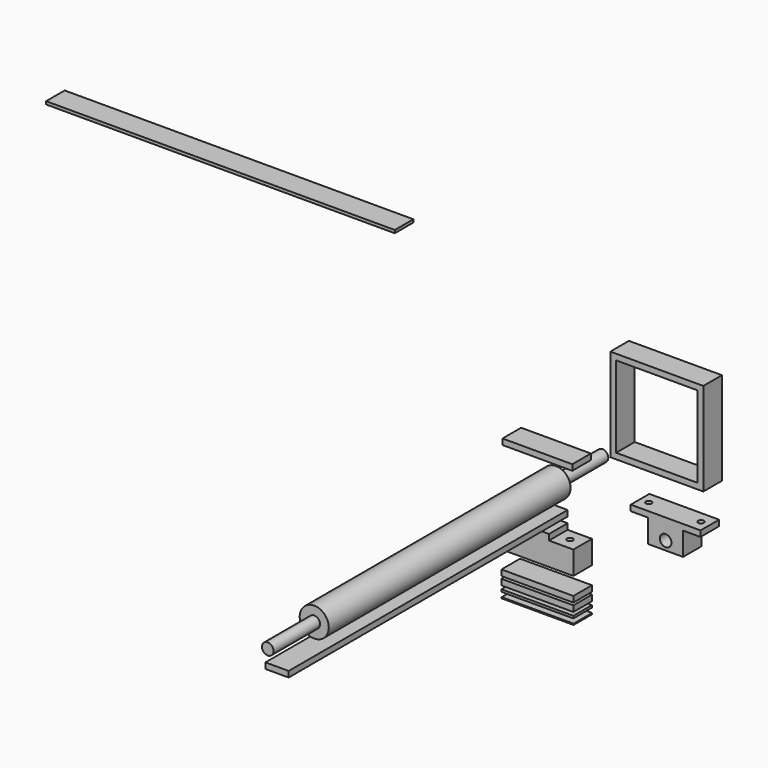
from build123d import *

# Parameters (mm, degrees)
F0_R      = 5
F1_DEPTH  = 20
F0_W      = 60
F0_H      = 5
F0_W_2    = 80
F0_H_2    = 80
F0_W_3    = 70
F0_H_3    = 70
F0_W_4    = 61.861140081
F0_H_4    = 1
F0_H_5    = 2
F0_W_5    = 300
F0_H_6    = 2.5
F0_R_2    = 12.5
F2_DEPTH  = 260
F3_R      = 5
F4_DEPTH  = 50
F5_DEPTH  = 300
F6_R      = 2.5
F7_R      = 2.5
F8_DEPTH  = 25
F10_R     = 2.5
F9_R      = 2.5
F11_DEPTH = 25
F17_R     = 5
F18_DEPTH = 50


# Not quite as in the source:
# - a feature of the source that left no trace in its solid (it failed there, or was rolled back) is left out
# - a feature names something its author has since deleted; it is built from what else it names


with BuildPart() as f1:
    # F0 (on Front) → F1 (new body)
    with BuildSketch(Plane.XZ):
        Polygon((95.2936565876, -7.5), (110.2936565876, -7.5), (125.2936565876, -7.5), (125.2936565876, 12.5), (140.2936565876, 12.5), (140.2936565876, 17.5), (110.2936565876, 17.5), (80.2936565876, 17.5), (80.2936565876, 12.5), (95.2936565876, 12.5), align=None)
        with Locations((110.2936565876, 0)):
            Circle(F0_R, mode=Mode.SUBTRACT)
    extrude(amount=F1_DEPTH)

    # F10 (on face) + F9 (on face) → F11 (cut)
    with BuildSketch(Plane(origin=(0, 0, 12.5), x_dir=(1, 0, 0), z_dir=(0, 0, -1))):
        with Locations((87.7936565876, 10)):
            Circle(F10_R)
    with BuildSketch(Plane(origin=(0, 0, 12.5), x_dir=(1, 0, 0), z_dir=(0, 0, -1))):
        with Locations((132.7936565876, 10)):
            Circle(F9_R)
    extrude(amount=-F11_DEPTH, mode=Mode.SUBTRACT)


with BuildPart() as f1b:
    # F0 (on Front) → F1, piece 2 (new body)
    with BuildSketch(Plane.XZ):
        with Locations((0, 29.2427036911)):
            Rectangle(F0_W, F0_H)
    extrude(amount=F1_DEPTH)


with BuildPart() as f1c:
    # F0 (on Front) → F1, piece 3 (new body)
    with BuildSketch(Plane.XZ):
        Polygon((10, -27.5771580637), (0, -27.5771580637), (-10, -27.5771580637), (-10, -32.5771580637), (-10.9305700405, -32.5771580637), (-30.9305700405, -32.5771580637), (-30.9305700405, -52.5771580637), (0, -52.5771580637), (30.9305700405, -52.5771580637), (30.9305700405, -32.5771580637), (10.9305700405, -32.5771580637), (10, -32.5771580637), align=None)
    extrude(amount=F1_DEPTH)

    # F6 (on face) + F7 (on face) → F8 (cut)
    with BuildSketch(Plane.XY.offset(-32.5771580637)):
        with Locations((-20, -10)):
            Circle(F6_R)
    with BuildSketch(Plane.XY.offset(-32.5771580637)):
        with Locations((20, -10)):
            Circle(F7_R)
    extrude(amount=-F8_DEPTH, mode=Mode.SUBTRACT)


with BuildPart() as f1d:
    # F0 (on Front) → F1, piece 4 (new body)
    with BuildSketch(Plane.XZ):
        with Locations((102.7326732874, 87.7068325877)):
            Rectangle(F0_W_2, F0_H_2)
        with Locations((102.7326732874, 87.7068325877)):
            Rectangle(F0_W_3, F0_H_3, mode=Mode.SUBTRACT)
    extrude(amount=F1_DEPTH)


with BuildPart() as f1e:
    # F0 (on Front) → F1, piece 5 (new body)
    with BuildSketch(Plane.XZ):
        with Locations((0, -77.355325222)):
            Rectangle(F0_W_4, F0_H)
    extrude(amount=F1_DEPTH)


with BuildPart() as f1f:
    # F0 (on Front) → F1, piece 6 (new body)
    with BuildSketch(Plane.XZ):
        with Locations((0.1928325291, -89.1451310813)):
            Rectangle(F0_W_4, F0_H_4)
    extrude(amount=F1_DEPTH)


with BuildPart() as f1g:
    # F0 (on Front) → F1, piece 7 (new body)
    with BuildSketch(Plane.XZ):
        with Locations((0, -83.756296128)):
            Rectangle(F0_W_4, F0_H_5)
    extrude(amount=F1_DEPTH)


with BuildPart() as f1h:
    # F0 (on Front) → F1, piece 8 (new body)
    with BuildSketch(Plane.XZ):
        with Locations((0, -70.2389810979)):
            Rectangle(F0_W_4, F0_H)
    extrude(amount=F1_DEPTH)


with BuildPart() as f1i:
    # F0 (on Front) → F1, piece 9 (new body)
    with BuildSketch(Plane.XZ):
        with Locations((-272.7023124695, 158.2453411818)):
            Rectangle(F0_W_5, F0_H_6)
    extrude(amount=F1_DEPTH)


with BuildPart() as f2:
    # F0 (on Front) → F2 (new body)
    with BuildSketch(Plane.XZ):
        Circle(F0_R_2)
    extrude(amount=F2_DEPTH)

    # F3 (on face) → F4 (join)
    with BuildSketch(Plane.XZ.offset(260)):
        Circle(F3_R)
    extrude(amount=F4_DEPTH)

    # F17 (on face) → F18 (join)
    with BuildSketch(Plane(origin=(0, 0, 0), x_dir=(-1, 0, 0), z_dir=(0, 1, 0))):
        Circle(F17_R)
    extrude(amount=F18_DEPTH)


with BuildPart() as f5:
    # F0 (on Front) → F5 (new body)
    with BuildSketch(Plane.XZ):
        Polygon((-10, -22.5167013705), (0, -22.5167013705), (10, -22.5167013705), (10, -17.5167013705), (0, -17.5167013705), (-10, -17.5167013705), align=None)
    extrude(amount=F5_DEPTH)


solid = Compound([f1.part, f1b.part, f1c.part, f1d.part, f1e.part, f1f.part, f1g.part, f1h.part, f1i.part, f2.part, f5.part])
